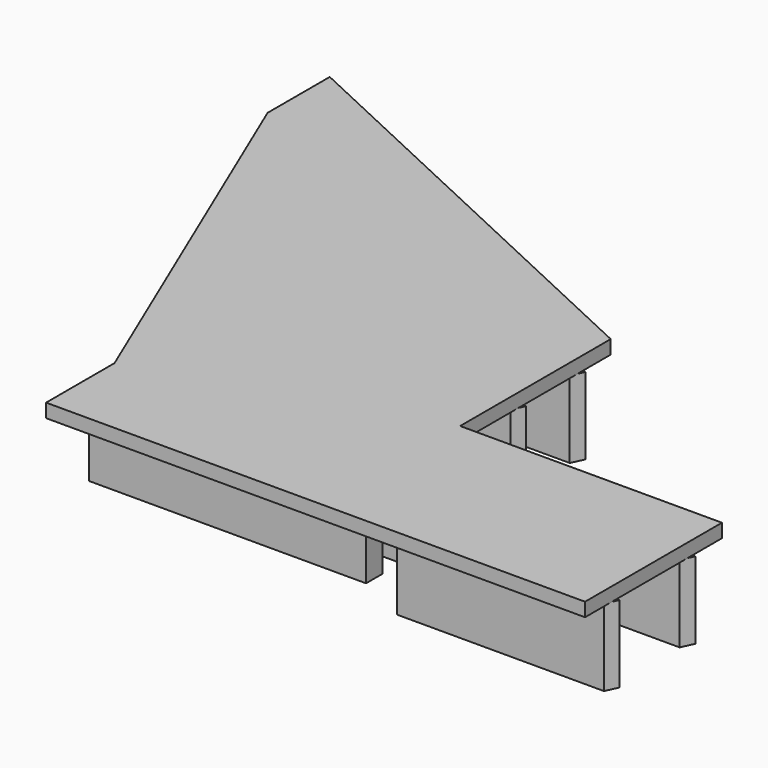
from build123d import *

# Parameters (mm, degrees)
F0_W     = 16.2
F0_H     = 1.2
F1_DEPTH = 4.5
F2_W     = 16.2
F2_H     = 0.675
F2_H_2   = 1.2
F2_H_3   = 3.125
F3_DEPTH = 0.8
F5_E28_W = 22.0063713977
F5_E28_H = 4.5
F5_E29_W = 12.0937982574
F5_E29_H = 4.5
F5_E30_W = 12.0937982574
F5_E30_H = 4.5
F5_E31_W = 11.5652361646
F5_E31_H = 4.5
F5_E32_W = 11.5652361646
F5_E32_H = 4.5
F6_DEPTH = 0.4


with BuildPart() as f1:
    # F0 (on Top) → F1 (new body)
    with BuildSketch(Plane.XY):
        with Locations((-29.7626322135, 18.7695161968)):
            Rectangle(F0_W, F0_H)
    extrude(amount=F1_DEPTH)



with BuildPart() as f1b:
    # F0 (on Top) → F1, piece 2 (new body)
    with BuildSketch(Plane.XY):
        with Locations((-29.7626322135, 16.2195161968)):
            Rectangle(F0_W, F0_H)
    extrude(amount=F1_DEPTH)


with BuildPart() as f1_1:
    add(f1.part)

    add(f1b.part)  # F3 merges F1b
    # F2 (on face) → F3 (join)
    with BuildSketch(Plane.XY.offset(4.5)):
        Polygon((-47.8626322135, 41.1793105304), (-37.8626322135, 17.4945161968), (-21.6626322135, 17.4945161968), (-21.6626322135, 22.4945161968), (-21.6626322135, 33.4945161968), (-47.8626322135, 45.7203537226), align=None)
        Polygon((-21.6626322135, 22.4945161968), (-21.6626322135, 17.4945161968), (-21.6626322135, 16.8195161968), (-21.6626322135, 15.6195161968), (-21.6626322135, 12.4945161968), (-6.3626514748, 12.4945161968), (-6.3626514748, 22.4945161968), align=None)
        with Locations((-29.7626322135, 17.1570161968)):
            Rectangle(F2_W, F2_H)
        with Locations((-29.7626322135, 16.2195161968)):
            Rectangle(F2_W, F2_H_2)
        with Locations((-29.7626322135, 14.0570161968)):
            Rectangle(F2_W, F2_H_3)
    extrude(amount=F3_DEPTH)

    # F5_E28 (on explicit) + F5_E29 (on explicit) + F5_E30 (on explicit) + F5_E31 (on explicit) + F5_E32 (on explicit) → F6 (join, symmetric)
    with BuildSketch(Plane(origin=(-47.8626322135, 43.4498321265, 4.5), x_dir=(0.9061941294, -0.4228619158, 0), z_dir=(0.4228619158, 0.9061941294, 0))):
        with Locations((11.0031856988, 2.25)):
            Rectangle(F5_E28_W, F5_E28_H)
    with BuildSketch(Plane(origin=(-18.4564497322, 19.9771542102, 4.5), x_dir=(1, 0, 0), z_dir=(0, 1, 0))):
        with Locations((6.0468991287, 2.25)):
            Rectangle(F5_E29_W, F5_E29_H)
    with BuildSketch(Plane(origin=(-18.4564497322, 14.4476536661, 4.5), x_dir=(1, 0, 0), z_dir=(0, 1, 0))):
        with Locations((6.0468991287, 2.25)):
            Rectangle(F5_E30_W, F5_E30_H)
    with BuildSketch(Plane(origin=(-21.6626322135, 31.073756516, 4.5), x_dir=(-1, 0, 0), z_dir=(0, -1, 0))):
        with Locations((5.7826180823, 2.25)):
            Rectangle(F5_E31_W, F5_E31_H)
    with BuildSketch(Plane(origin=(-21.6626322135, 26.7479624599, 4.5), x_dir=(-1, 0, 0), z_dir=(0, -1, 0))):
        with Locations((5.7826180823, 2.25)):
            Rectangle(F5_E32_W, F5_E32_H)
    extrude(amount=F6_DEPTH, both=True, dir=(0.4228619158, 0.9061941294, 0))


solid = f1_1.part
